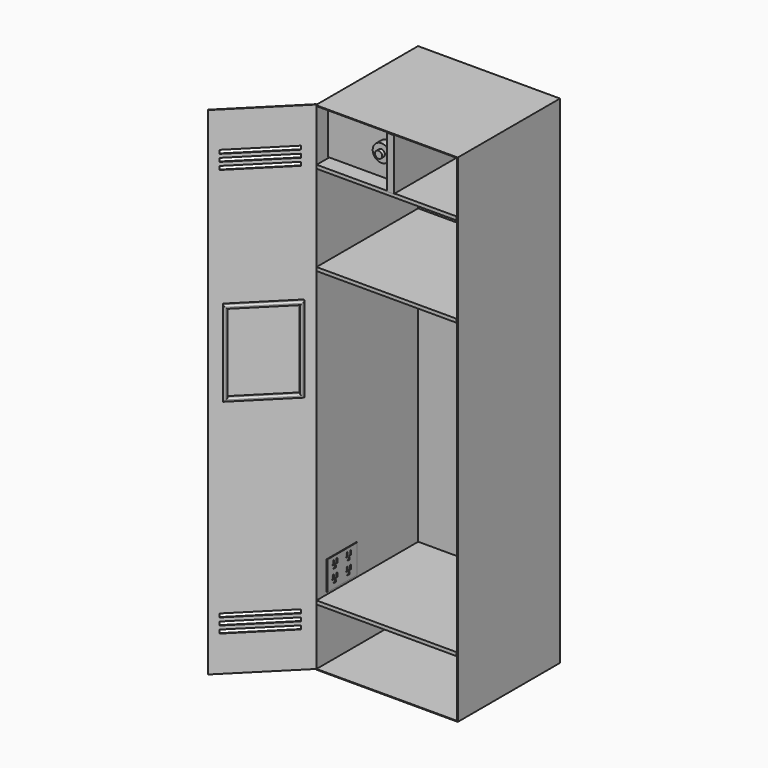
from build123d import *

# Parameters (mm, degrees)
F0_W      = 508
F0_H      = 1778
F1_DEPTH  = 457.2
F2_T      = -2.54
F5_W      = 304.8
F5_H      = 1778
F5_W_2    = 228.6
F5_H_2    = 12.7
F6_DEPTH  = 2.54
F7_W      = 50.8
F7_H      = 101.6
F8_DEPTH  = 25.4
F10_W     = 501.142
F10_H     = 12.7
F10_W_2   = 501.9836910069
F12_R     = 8.89
F13_DEPTH = 502.92
F14_W     = 228.6
F14_H     = 304.8
F14_W_2   = 203.2
F14_H_2   = 279.4
F15_DEPTH = 12.7
F16_R     = 5.08
F17_W     = 12.7
F17_H     = 180.5464800811
F18_DEPTH = 254
F19_R     = 31.0325026996
F20_DEPTH = 25.4
F21_R     = 12.7
F22_DEPTH = 12.7
F23_W     = 50.8
F23_H     = 44.1827178001
F24_DEPTH = 7.62
F25_W     = 133.1598460674
F25_H     = 103.0222028494
F26_DEPTH = 2.54
F27_W     = 7.4603557587
F27_H     = 7.4603557587
F28_DEPTH = 7.62
F29_R     = 1.27
F30_W     = 453.6709259264
F30_H     = 185.0115060806
F31_DEPTH = 25.4
F32_W     = 7.62
F32_H     = 15.24
F33_DEPTH = 2.54


# Not quite as in the source:
# - a feature names something its author has since deleted; it is built from what else it names


with BuildPart() as f1:
    # F0 (on Front) → F1 (new body)
    with BuildSketch(Plane.XZ):
        with Locations((225.2186250836, 819.9913739562)):
            Rectangle(F0_W, F0_H)
    extrude(amount=F1_DEPTH)

    # F2
    f2_openings = [f1.faces().sort_by_distance(p)[0] for p in [
        (225.218625, -457.2, 819.991374),
    ]]
    offset(amount=F2_T, openings=f2_openings)

    # F5 (on face) → F6 (join)
    with BuildSketch(Plane(origin=(215.4793125418, -215.4793125418, 0), x_dir=(-0.7071067812, -0.7071067812, 0), z_dir=(-0.7071067812, 0.7071067812, 0))):
        with Locations((494.2344263691, 822.4811866283)):
            Rectangle(F5_W, F5_H)
        with Locations((499.739182663, 66.8311866283)):
            Rectangle(F5_W_2, F5_H_2, mode=Mode.SUBTRACT)
        with Locations((499.739182663, 92.2311866283)):
            Rectangle(F5_W_2, F5_H_2, mode=Mode.SUBTRACT)
        with Locations((499.739182663, 117.6311866283)):
            Rectangle(F5_W_2, F5_H_2, mode=Mode.SUBTRACT)
        with Locations((499.739182663, 1527.3311866283)):
            Rectangle(F5_W_2, F5_H_2, mode=Mode.SUBTRACT)
        with Locations((499.739182663, 1552.7311866283)):
            Rectangle(F5_W_2, F5_H_2, mode=Mode.SUBTRACT)
        with Locations((499.739182663, 1578.1311866283)):
            Rectangle(F5_W_2, F5_H_2, mode=Mode.SUBTRACT)
    extrude(amount=F6_DEPTH)

    # F7 (on face) → F8 (join)
    with BuildSketch(Plane(origin=(213.6832613176, -213.6832613176, 0), x_dir=(-0.7071067812, -0.7071067812, 0), z_dir=(-0.7071067812, 0.7071067812, 0))):
        with Locations((577.3518989235, 900.0128252983)):
            Rectangle(F7_W, F7_H)
    extrude(amount=F8_DEPTH)

    # F10 (on offset) → F11 (join, up to the next surface of F1)
    with BuildSketch(Plane.XZ.offset(457.2)):
        with Locations((224.3739893488, 143.0813739562)):
            Rectangle(F10_W, F10_H)
        with Locations((224.3921216577, 1193.3354927063)):
            Rectangle(F10_W_2, F10_H)
        with Locations((224.8129671612, 1515.6838489532)):
            Rectangle(F10_W, F10_H)
    extrude(until=Until.NEXT, dir=(0, 1, 0))

    # F12 (on face) → F13 (join, through all)
    with BuildSketch(Plane(origin=(476.6786250836, 0, 0), x_dir=(0, -1, 0), z_dir=(-1, 0, 0))):
        with Locations((253.790974617, 1154.0207862854)):
            Circle(F12_R)
    extrude(amount=F13_DEPTH)

    # F14 (on face) → F15 (join)
    with BuildSketch(Plane(origin=(215.4793125418, -215.4793125418, 0), x_dir=(0.7071067812, 0.7071067812, 0), z_dir=(0.7071067812, -0.7071067812, 0))):
        with Locations((-491.1756113548, 947.155437104)):
            Rectangle(F14_W, F14_H)
        with Locations((-491.1756113548, 947.155437104)):
            Rectangle(F14_W_2, F14_H_2, mode=Mode.SUBTRACT)
    extrude(amount=F15_DEPTH)

    # F16
    f16_edges = [f1.edges().sort_by_distance(p)[0] for p in [
        (-203.676342, -652.595479, 947.155437),
        (-122.854037, -571.773174, 1099.555437),
        (-42.031732, -490.950869, 947.155437),
        (-122.854037, -571.773174, 794.755437),
        (-122.854037, -571.773174, 807.455437),
        (-51.011988, -499.931125, 947.155437),
        (-194.696086, -643.615223, 947.155437),
        (-122.854037, -571.773174, 1086.855437),
    ]]
    fillet(f16_edges, radius=F16_R)

    # F17 (on face) → F18 (join)
    with BuildSketch(Plane.YZ.offset(-26.2413749164)):
        with Locations((-400.0427534704, 1616.1781339157)):
            Rectangle(F17_W, F17_H)
    extrude(amount=F18_DEPTH)

    # F19 (on face) → F20 (join)
    with BuildSketch(Plane.XZ.offset(406.3927534704)):
        with Locations((185.4707747698, 1617.2170639038)):
            Circle(F19_R)
    extrude(amount=F20_DEPTH)

    # F21 (on face) → F22 (join)
    with BuildSketch(Plane.XZ.offset(431.7927534704)):
        with Locations((185.4707747698, 1617.2170639038)):
            Circle(F21_R)
    extrude(amount=F22_DEPTH)

    # F23 (on face) → F24 (join)
    with BuildSketch(Plane(origin=(195.7227490754, -195.7227490754, 0), x_dir=(-0.7071067812, -0.7071067812, 0), z_dir=(-0.7071067812, 0.7071067812, 0))):
        with BuildLine():
            add(Edge.make_bspline(
                [(576.0113596916, 944.98026371), (551.8075273357, 944.98026371), (563.9094435137, 913.3750796318), (576.0113596916, 881.7698955536), (588.1132758696, 913.3750796318), (600.2151920475, 944.98026371), (576.0113596916, 944.98026371)],
                knots=[0, 0, 0, 2.0943951024, 2.0943951024, 4.1887902048, 4.1887902048, 6.2831853072, 6.2831853072, 6.2831853072], degree=2, weights=[1, 0.5, 1, 0.5, 1, 0.5, 1]))
        make_face()
        with Locations((577.3518989235, 871.3041841984)):
            Rectangle(F23_W, F23_H)
    extrude(amount=F24_DEPTH)

    # F25 (on face) → F26 (join)
    with BuildSketch(Plane.YZ.offset(-26.2413749164)):
        with Locations((-345.3890532255, 209.1637179255)):
            Rectangle(F25_W, F25_H)
    extrude(amount=F26_DEPTH)

    # F27 (on face) → F28 (join)
    with BuildSketch(Plane(origin=(190.3345954028, -190.3345954028, 0), x_dir=(-0.7071067812, -0.7071067812, 0), z_dir=(-0.7071067812, 0.7071067812, 0))):
        with Locations((562.4311566353, 881.6170096397)):
            Rectangle(F27_W, F27_H)
        with Locations((576.0353207588, 881.6170096397)):
            Rectangle(F27_W, F27_H)
        with Locations((590.0784134865, 881.6170096397)):
            Rectangle(F27_W, F27_H)
        with Locations((562.4311566353, 870.6458210945)):
            Rectangle(F27_W, F27_H)
        with Locations((576.0353207588, 870.6458210945)):
            Rectangle(F27_W, F27_H)
        with Locations((590.0784134865, 870.6458210945)):
            Rectangle(F27_W, F27_H)
        with Locations((562.4311566353, 859.6748709679)):
            Rectangle(F27_W, F27_H)
        with Locations((576.0353207588, 859.6748709679)):
            Rectangle(F27_W, F27_H)
        with Locations((590.0784134865, 859.6748709679)):
            Rectangle(F27_W, F27_H)
    extrude(amount=F28_DEPTH)

    # F29
    f29_edges = [f1.edges().sort_by_distance(p)[0] for p in [
        (-212.752443, -582.645327, 885.347188),
        (-210.114809, -580.007692, 881.61701),
        (-212.752443, -582.645327, 877.886832),
        (-215.390077, -585.282961, 881.61701),
        (-222.37204, -592.264923, 877.886832),
        (-225.009674, -594.902557, 881.61701),
        (-222.37204, -592.264923, 885.347188),
        (-219.734406, -589.627289, 881.61701),
        (-232.302006, -602.194889, 885.347188),
        (-229.664372, -599.557255, 881.61701),
        (-232.302006, -602.194889, 877.886832),
        (-234.93964, -604.832523, 881.61701),
        (-229.664372, -599.557255, 870.645821),
        (-232.302006, -602.194889, 866.915643),
        (-234.93964, -604.832523, 870.645821),
        (-232.302006, -602.194889, 874.375999),
        (-222.37204, -592.264923, 866.915643),
        (-225.009674, -594.902557, 870.645821),
        (-222.37204, -592.264923, 874.375999),
        (-219.734406, -589.627289, 870.645821),
        (-212.752443, -582.645327, 874.375999),
        (-210.114809, -580.007692, 870.645821),
        (-212.752443, -582.645327, 866.915643),
        (-215.390077, -585.282961, 870.645821),
        (-212.752443, -582.645327, 863.405049),
        (-210.114809, -580.007692, 859.674871),
        (-212.752443, -582.645327, 855.944693),
        (-215.390077, -585.282961, 859.674871),
        (-222.37204, -592.264923, 855.944693),
        (-225.009674, -594.902557, 859.674871),
        (-222.37204, -592.264923, 863.405049),
        (-219.734406, -589.627289, 859.674871),
        (-234.93964, -604.832523, 859.674871),
        (-232.302006, -602.194889, 863.405049),
        (-229.664372, -599.557255, 859.674871),
        (-232.302006, -602.194889, 855.944693),
        (-207.420732, -582.701769, 855.944693),
        (-207.420732, -582.701769, 863.405049),
        (-212.696, -587.977037, 855.944693),
        (-217.040329, -592.321366, 855.944693),
        (-217.040329, -592.321366, 863.405049),
        (-217.040329, -592.321366, 866.915643),
        (-217.040329, -592.321366, 874.375999),
        (-217.040329, -592.321366, 877.886832),
        (-217.040329, -592.321366, 885.347188),
        (-207.420732, -582.701769, 866.915643),
        (-207.420732, -582.701769, 874.375999),
        (-207.420732, -582.701769, 877.886832),
        (-207.420732, -582.701769, 885.347188),
        (-222.315597, -597.596634, 877.886832),
        (-222.315597, -597.596634, 866.915643),
        (-212.696, -587.977037, 866.915643),
        (-222.315597, -597.596634, 855.944693),
        (-226.970295, -602.251332, 855.944693),
        (-226.970295, -602.251332, 863.405049),
        (-226.970295, -602.251332, 866.915643),
        (-226.970295, -602.251332, 874.375999),
        (-226.970295, -602.251332, 877.886832),
        (-226.970295, -602.251332, 885.347188),
        (-232.245563, -607.5266, 855.944693),
        (-232.245563, -607.5266, 866.915643),
        (-232.245563, -607.5266, 877.886832),
        (-232.245563, -607.5266, 885.347188),
        (-232.245563, -607.5266, 874.375999),
        (-232.245563, -607.5266, 863.405049),
        (-222.315597, -597.596634, 863.405049),
        (-222.315597, -597.596634, 874.375999),
        (-222.315597, -597.596634, 885.347188),
        (-212.696, -587.977037, 885.347188),
        (-212.696, -587.977037, 874.375999),
        (-212.696, -587.977037, 863.405049),
    ]]
    fillet(f29_edges, radius=F29_R)

    # F30 (on face) → F31 (join)
    with BuildSketch(Plane.YZ.offset(227.7586250836)):
        with Locations((-233.3540881518, 1614.2709851265)):
            Rectangle(F30_W, F30_H)
    extrude(amount=F31_DEPTH)

    # F32 (on face) → F33 (cut)
    with BuildSketch(Plane.YZ.offset(-23.7013749164)):
        with Locations((-386.169571104, 239.9441816854)):
            Rectangle(F32_W, F32_H)
        with Locations((-370.929571104, 239.9441816854)):
            Rectangle(F32_W, F32_H)
        with BuildLine():
            ThreePointArc((-373.469571104, 224.7041816854), (-378.549571104, 229.7841816854), (-383.629571104, 224.7041816854))
            Line((-383.629571104, 224.7041816854), (-383.629571104, 219.7599632359))
            Line((-383.629571104, 219.7599632359), (-373.469571104, 219.7599632359))
            Line((-373.469571104, 219.7599632359), (-373.469571104, 224.7041816854))
        make_face()
        with Locations((-325.209571104, 239.9441816854)):
            Rectangle(F32_W, F32_H)
        with Locations((-309.969571104, 239.9441816854)):
            Rectangle(F32_W, F32_H)
        with BuildLine():
            Line((-322.669571104, 224.7041816854), (-322.669571104, 219.7599632359))
            Line((-322.669571104, 219.7599632359), (-312.509571104, 219.7599632359))
            Line((-312.509571104, 219.7599632359), (-312.509571104, 224.7041816854))
            ThreePointArc((-312.509571104, 224.7041816854), (-317.589571104, 229.7841816854), (-322.669571104, 224.7041816854))
        make_face()
        with Locations((-386.4056682646, 194.4787946957)):
            Rectangle(F32_W, F32_H)
        with BuildLine():
            ThreePointArc((-373.7056682646, 179.2387946957), (-378.7856682646, 184.3187946957), (-383.8656682646, 179.2387946957))
            Line((-383.8656682646, 179.2387946957), (-383.8656682646, 174.2945762461))
            Line((-383.8656682646, 174.2945762461), (-373.7056682646, 174.2945762461))
            Line((-373.7056682646, 174.2945762461), (-373.7056682646, 179.2387946957))
        make_face()
        with Locations((-371.1656682646, 194.4787946957)):
            Rectangle(F32_W, F32_H)
        with Locations((-325.6173620766, 194.4800104896)):
            Rectangle(F32_W, F32_H)
        with Locations((-310.3773620766, 194.4800104896)):
            Rectangle(F32_W, F32_H)
        with BuildLine():
            Line((-312.9173620766, 174.29579204), (-312.9173620766, 179.2400104896))
            ThreePointArc((-312.9173620766, 179.2400104896), (-317.9973620766, 184.3200104896), (-323.0773620766, 179.2400104896))
            Line((-323.0773620766, 179.2400104896), (-323.0773620766, 174.29579204))
            Line((-323.0773620766, 174.29579204), (-312.9173620766, 174.29579204))
        make_face()
    extrude(amount=-F33_DEPTH, mode=Mode.SUBTRACT)


solid = f1.part
